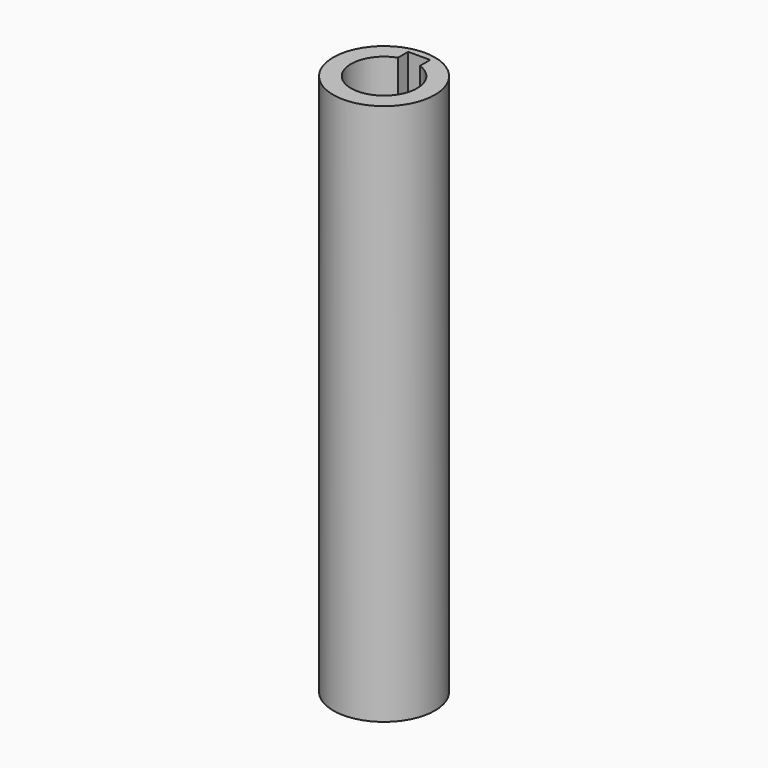
from build123d import *

# Parameters (mm, degrees)
F0_R     = 15
F1_DEPTH = 160
F3_DEPTH = 40


# Not quite as in the source:
# - a feature names something its author has since deleted; it is built from what else it names


with BuildPart() as f1:
    # F0 (on Top) → F1 (new body)
    with BuildSketch(Plane.XY):
        Circle(F0_R)
    extrude(amount=F1_DEPTH)

    # F2 (on face) → F3 (cut)
    with BuildSketch(Plane.XY.offset(160)):
        with BuildLine():
            ThreePointArc((-3.25, 9.1923881554), (-5.6291651246, -7.960841664), (9.75, 0))
            ThreePointArc((9.75, 0), (7.960841664, 5.6291651246), (3.25, 9.1923881554))
            Line((3.25, 9.1923881554), (3.25, 6.55))
            Line((3.25, 6.55), (-3.25, 6.55))
            Line((-3.25, 6.55), (-3.25, 9.1923881554))
        make_face()
        with BuildLine():
            Line((3.25, 6.55), (3.25, 9.1923881554))
            ThreePointArc((3.25, 9.1923881554), (0, 9.75), (-3.25, 9.1923881554))
            Line((-3.25, 9.1923881554), (-3.25, 6.55))
            Line((-3.25, 6.55), (3.25, 6.55))
        make_face()
        with BuildLine():
            ThreePointArc((-3.25, 9.1923881554), (0, 9.75), (3.25, 9.1923881554))
            Line((3.25, 9.1923881554), (3.25, 12.95))
            Line((3.25, 12.95), (-3.25, 12.95))
            Line((-3.25, 12.95), (-3.25, 9.1923881554))
        make_face()
    extrude(amount=-F3_DEPTH, mode=Mode.SUBTRACT)


solid = f1.part
